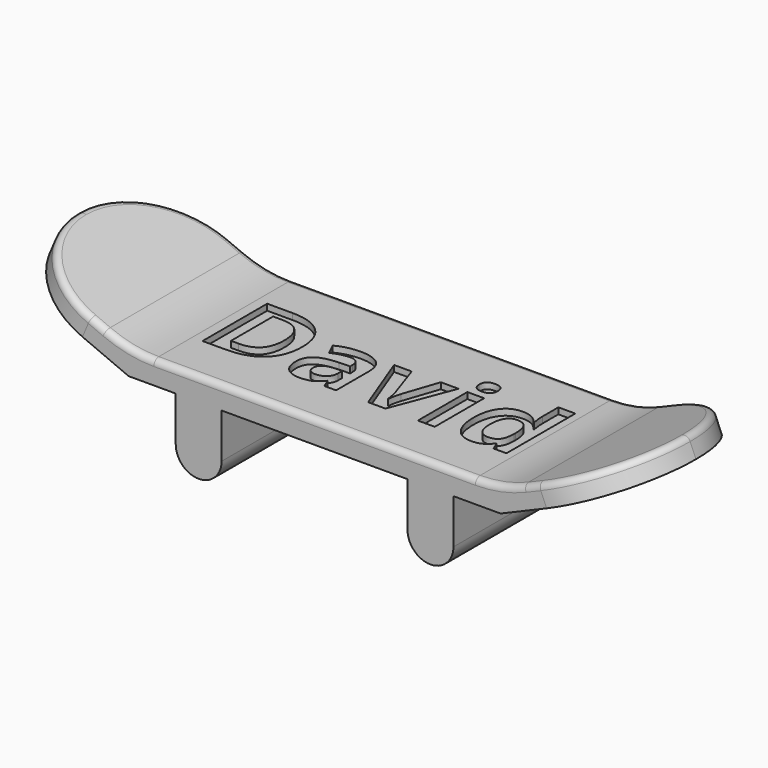
from build123d import *

# Parameters (mm, degrees)
F1_DEPTH     = 28
F2_R         = 13.99999
F3_R         = 20
F4_T1_DEPTH  = 51.8619080231
F4_T3_DEPTH  = 2.5763226316
F4_T5_DEPTH  = 2e-05
F4_T7_DEPTH  = 2.5763226316
F4_T10_ANGLE = 90
F4_T12_ANGLE = 90
F4_T14_ANGLE = 23
F4_T16_ANGLE = 23
F4_T18_ANGLE = 23
F4_T20_ANGLE = 23
F4_T22_ANGLE = 90
F4_T24_ANGLE = 90
F5_TEXT_SIZE = 18.2712876444
F6_DEPTH     = 1


# Not quite as in the source:
# - a fillet or chamfer that OpenCascade refuses, or shapes differently, is made with other operations: its cross-section is extruded or revolved along the edge and cut away or added
# - a fillet or chamfer is up to 0.001 mm smaller than in the source, because OpenCascade refuses the exact size
# - Text() gives the source's letters only with a copy of the font that has no kerning and outlines rounded to 1/6400 em; it was checked with that copy


with BuildPart() as f1:
    # F0 (on Front) → F1 (new body)
    with BuildSketch(Plane.XZ):
        Polygon((-15, 0), (0, 0), (15, 0), (22.4, 0), (30, 0), (50.3326386479, 8.6306930531), (49.0041528111, 11.7604095549), (30, 3.6936252832), (0, 3.6936252832), (-30, 3.6936252832), (-49.0041528111, 11.7604095549), (-50.3326386479, 8.6306930531), (-30, 0), (-22.4, 0), align=None)
        with BuildLine():
            Line((-15, -7.2063747168), (-15, 0))
            Line((-15, 0), (-22.4, 0))
            Line((-22.4, 0), (-22.4, -7.2063747168))
            ThreePointArc((-22.4, -7.2063747168), (-18.7, -10.9063747168), (-15, -7.2063747168))
        make_face()
        with BuildLine():
            Line((22.4, 0), (15, 0))
            Line((15, 0), (15, -7.2063747168))
            ThreePointArc((15, -7.2063747168), (18.7, -10.9063747168), (22.4, -7.2063747168))
            Line((22.4, -7.2063747168), (22.4, 0))
        make_face()
    extrude(amount=F1_DEPTH)

    # F2 (radius 14 in the source; OpenCascade refuses exactly that, so slightly less here)
    f2_edges = [f1.edges().sort_by_distance(p)[0] for p in [
        (49.668396, 0, 10.195551),
        (49.668396, -28, 10.195551),
        (-49.668396, 0, 10.195551),
        (-49.668396, -28, 10.195551),
    ]]
    fillet(f2_edges, radius=F2_R)

    # F3
    f3_edges = [f1.edges().sort_by_distance(p)[0] for p in [
        (30, -14, 3.693625),
        (-30, -14, 3.693625),
    ]]
    fillet(f3_edges, radius=F3_R)

    # F4: fillet of radius 1 on 18 edges, made by hand

    # F4_s2 → F4_t1 (cut)
    with BuildSketch(Plane.YZ.offset(-25.9309540115)):
        with BuildLine():
            ThreePointArc((0, 2.6936252832), (-0.2928932188, 3.4007320644), (-1, 3.6936252832))
            Line((-1, 3.6936252832), (0, 3.6936252832))
            Line((0, 3.6936252832), (0, 2.6936252832))
        make_face()
        with BuildLine():
            ThreePointArc((-28, 2.6936252832), (-27.7071067812, 3.4007320644), (-27, 3.6936252832))
            Line((-27, 3.6936252832), (-28, 3.6936252832))
            Line((-28, 3.6936252832), (-28, 2.6936252832))
        make_face()
    extrude(amount=F4_T1_DEPTH, mode=Mode.SUBTRACT)

    # F4_s4 → F4_t3 (cut)
    with BuildSketch(Plane(origin=(-30.4939379751, 0, 12.9439087175), x_dir=(0, 1, 0), z_dir=(-0.9205048535, 0, 0.3907311285))):
        with BuildLine():
            ThreePointArc((-1, 8.3219338547), (-0.2928932188, 8.6148270735), (0, 9.3219338547))
            Line((0, 9.3219338547), (0, 8.3219338547))
            Line((0, 8.3219338547), (-1, 8.3219338547))
        make_face()
        with BuildLine():
            ThreePointArc((-27, 8.3219338547), (-27.7071067812, 8.6148270735), (-28, 9.3219338547))
            Line((-28, 9.3219338547), (-28, 8.3219338547))
            Line((-28, 8.3219338547), (-27, 8.3219338547))
        make_face()
    extrude(amount=F4_T3_DEPTH, mode=Mode.SUBTRACT)

    # F4_s6 → F4_t5 (cut)
    with BuildSketch(Plane.XZ.offset(13.99999)):
        with BuildLine():
            ThreePointArc((-48.0836479576, 11.3696784264), (-48.8489856795, 11.3763574275), (-49.3948839396, 10.8399047014))
            Line((-49.3948839396, 10.8399047014), (-49.0041528111, 11.7604095549))
            Line((-49.0041528111, 11.7604095549), (-48.0836479576, 11.3696784264))
        make_face()
        with BuildLine():
            ThreePointArc((48.0836479576, 11.3696784264), (48.8489856795, 11.3763574275), (49.3948839396, 10.8399047014))
            Line((49.3948839396, 10.8399047014), (49.0041528111, 11.7604095549))
            Line((49.0041528111, 11.7604095549), (48.0836479576, 11.3696784264))
        make_face()
    extrude(amount=F4_T5_DEPTH, mode=Mode.SUBTRACT)

    # F4_s8 → F4_t7 (cut)
    with BuildSketch(Plane(origin=(32.8654554615, 0, 13.9505581667), x_dir=(0, 1, 0), z_dir=(-0.9205048535, 0, -0.3907311285))):
        with BuildLine():
            ThreePointArc((0, 9.3219338547), (-0.2928932188, 8.6148270735), (-1, 8.3219338547))
            Line((-1, 8.3219338547), (0, 8.3219338547))
            Line((0, 8.3219338547), (0, 9.3219338547))
        make_face()
        with BuildLine():
            ThreePointArc((-28, 9.3219338547), (-27.7071067812, 8.6148270735), (-27, 8.3219338547))
            Line((-27, 8.3219338547), (-28, 8.3219338547))
            Line((-28, 8.3219338547), (-28, 9.3219338547))
        make_face()
    extrude(amount=F4_T7_DEPTH, mode=Mode.SUBTRACT)

    # F4_s9 → F4_t10 (revolve, cut)
    with BuildSketch(Plane.XZ.offset(13.99999)):
        with BuildLine():
            ThreePointArc((-48.0836479576, 11.3696784264), (-48.8489856795, 11.3763574275), (-49.3948839396, 10.8399047014))
            Line((-49.3948839396, 10.8399047014), (-49.0041528111, 11.7604095549))
            Line((-49.0041528111, 11.7604095549), (-48.0836479576, 11.3696784264))
        make_face()
    revolve(axis=Axis((-36.1170940678, -13.99999, 6.2901776633), (-0.3907311285, 0, -0.9205048535)), revolution_arc=F4_T10_ANGLE, mode=Mode.SUBTRACT)

    # F4_s11 → F4_t12 (revolve, cut)
    with BuildSketch(Plane.XZ.offset(14.00001)):
        with BuildLine():
            ThreePointArc((-48.0836479576, 11.3696784264), (-48.8489856795, 11.3763574275), (-49.3948839396, 10.8399047014))
            Line((-49.3948839396, 10.8399047014), (-49.0041528111, 11.7604095549))
            Line((-49.0041528111, 11.7604095549), (-48.0836479576, 11.3696784264))
        make_face()
    revolve(axis=Axis((-36.1170940678, -14.00001, 6.2901776633), (0.3907311285, 0, 0.9205048535)), revolution_arc=F4_T12_ANGLE, mode=Mode.SUBTRACT)

    # F4_s13 → F4_t14 (revolve, cut)
    with BuildSketch(Plane(origin=(-30.4939379751, 0, 12.9439087175), x_dir=(0, 1, 0), z_dir=(-0.9205048535, 0, 0.3907311285))):
        with BuildLine():
            ThreePointArc((0, 9.3219338547), (-0.2928932188, 8.6148270735), (-1, 8.3219338547))
            Line((-1, 8.3219338547), (0, 8.3219338547))
            Line((0, 8.3219338547), (0, 9.3219338547))
        make_face()
    revolve(axis=Axis((-25.9309540115, 0, 23.6936252832), (0, -1, 0)), revolution_arc=F4_T14_ANGLE, mode=Mode.SUBTRACT)

    # F4_s15 → F4_t16 (revolve, cut)
    with BuildSketch(Plane.YZ.offset(25.9309540115)):
        with BuildLine():
            ThreePointArc((0, 2.6936252832), (-0.2928932188, 3.4007320644), (-1, 3.6936252832))
            Line((-1, 3.6936252832), (0, 3.6936252832))
            Line((0, 3.6936252832), (0, 2.6936252832))
        make_face()
    revolve(axis=Axis((25.9309540115, 0, 23.6936252832), (0, -1, 0)), revolution_arc=F4_T16_ANGLE, mode=Mode.SUBTRACT)

    # F4_s17 → F4_t18 (revolve, cut)
    with BuildSketch(Plane(origin=(-30.4939379751, 0, 12.9439087175), x_dir=(0, 1, 0), z_dir=(-0.9205048535, 0, 0.3907311285))):
        with BuildLine():
            ThreePointArc((-27, 8.3219338547), (-27.7071067812, 8.6148270735), (-28, 9.3219338547))
            Line((-28, 9.3219338547), (-28, 8.3219338547))
            Line((-28, 8.3219338547), (-27, 8.3219338547))
        make_face()
    revolve(axis=Axis((-25.9309540115, -28, 23.6936252832), (0, -1, 0)), revolution_arc=F4_T18_ANGLE, mode=Mode.SUBTRACT)

    # F4_s19 → F4_t20 (revolve, cut)
    with BuildSketch(Plane.YZ.offset(25.9309540115)):
        with BuildLine():
            ThreePointArc((-28, 2.6936252832), (-27.7071067812, 3.4007320644), (-27, 3.6936252832))
            Line((-27, 3.6936252832), (-28, 3.6936252832))
            Line((-28, 3.6936252832), (-28, 2.6936252832))
        make_face()
    revolve(axis=Axis((25.9309540115, -28, 23.6936252832), (0, -1, 0)), revolution_arc=F4_T20_ANGLE, mode=Mode.SUBTRACT)

    # F4_s21 → F4_t22 (revolve, cut)
    with BuildSketch(Plane.XZ.offset(13.99999)):
        with BuildLine():
            ThreePointArc((48.0836479576, 11.3696784264), (48.8489856795, 11.3763574275), (49.3948839396, 10.8399047014))
            Line((49.3948839396, 10.8399047014), (49.0041528111, 11.7604095549))
            Line((49.0041528111, 11.7604095549), (48.0836479576, 11.3696784264))
        make_face()
    revolve(axis=Axis((36.1170940678, -13.99999, 6.2901776633), (-0.3907311285, 0, 0.9205048535)), revolution_arc=F4_T22_ANGLE, mode=Mode.SUBTRACT)

    # F4_s23 → F4_t24 (revolve, cut)
    with BuildSketch(Plane.XZ.offset(14.00001)):
        with BuildLine():
            ThreePointArc((48.0836479576, 11.3696784264), (48.8489856795, 11.3763574275), (49.3948839396, 10.8399047014))
            Line((49.3948839396, 10.8399047014), (49.0041528111, 11.7604095549))
            Line((49.0041528111, 11.7604095549), (48.0836479576, 11.3696784264))
        make_face()
    revolve(axis=Axis((36.1170940678, -14.00001, 6.2901776633), (0.3907311285, 0, -0.9205048535)), revolution_arc=F4_T24_ANGLE, mode=Mode.SUBTRACT)

    # F5 (on face) → F6 (cut)
    with BuildSketch(Plane.XY.offset(3.6936252832)):
        with Locations((-25.9309540115, -20.2377819474)):
            Text('David', F5_TEXT_SIZE, font='Open Sans', font_style=FontStyle.BOLD, text_align=(TextAlign.LEFT, TextAlign.BOTTOM))
    extrude(amount=-F6_DEPTH, mode=Mode.SUBTRACT)


solid = f1.part
